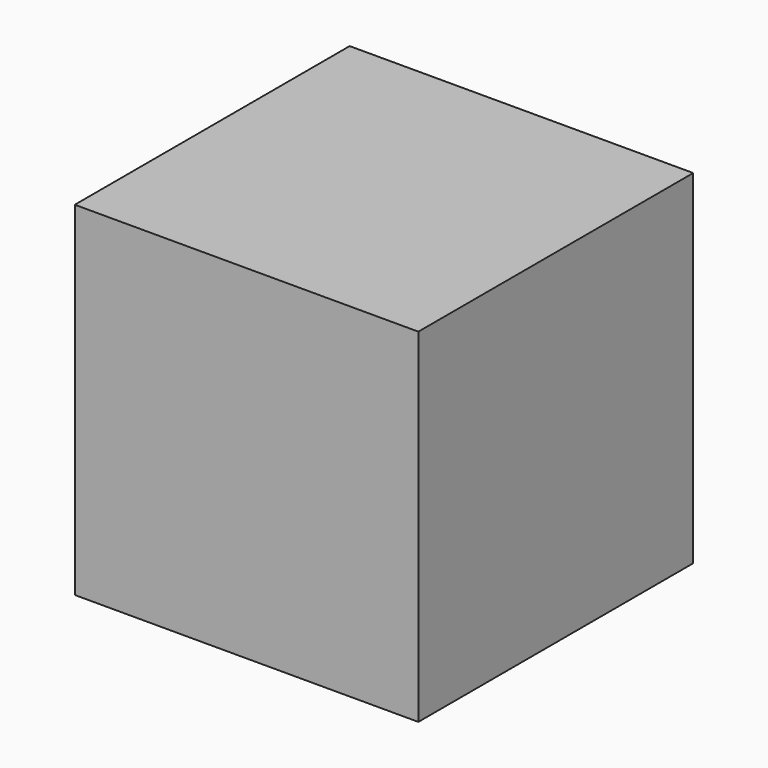
from build123d import *

# Parameters (mm, degrees)
F0_W          = 50
F0_H          = 50
F1_DEPTH      = 25
F1_DEPTH_BACK = 25


# Not quite as in the source:
# - the program builds the solid bodies; features that only make, move or delete a surface that nothing else refers to are left out


with BuildPart() as f1:
    # F0 (on Top) → F1 (new body, two sides)
    with BuildSketch(Plane.XY) as f1_sk:
        Rectangle(F0_W, F0_H)
    extrude(amount=F1_DEPTH)
    extrude(f1_sk.sketch, amount=-F1_DEPTH_BACK)


solid = f1.part
